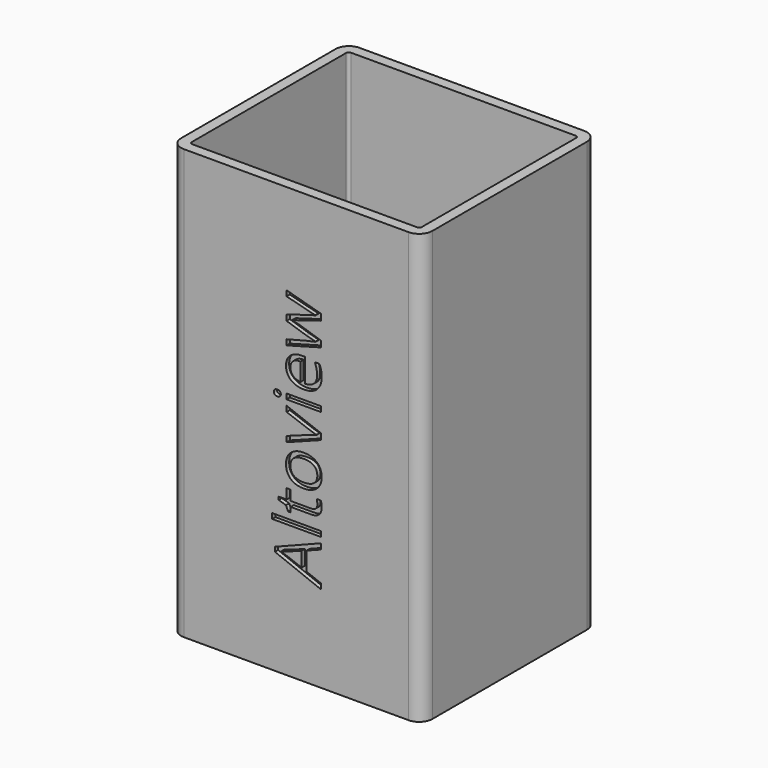
from build123d import *

# Parameters (mm, degrees)
F1_DEPTH     = 65
F2_T         = -1.6
F3_TEXT_SIZE = 9.7222222222
F4_DEPTH     = 0.6


# Not quite as in the source:
# - Text() gives the source's letters only with a copy of the font that has no kerning and outlines rounded to 1/6400 em; it was checked with that copy


with BuildPart() as f1:
    # F0 (on Top) → F1 (new body)
    with BuildSketch(Plane.XY):
        with BuildLine():
            Line((17, 16.6), (-17, 16.6))
            ThreePointArc((-17, 16.6), (-18.4142135624, 16.0142135624), (-19, 14.6))
            Line((-19, 14.6), (-19, -14.6))
            ThreePointArc((-19, -14.6), (-18.4142135624, -16.0142135624), (-17, -16.6))
            Line((-17, -16.6), (17, -16.6))
            ThreePointArc((17, -16.6), (18.4142135624, -16.0142135624), (19, -14.6))
            Line((19, -14.6), (19, 14.6))
            ThreePointArc((19, 14.6), (18.4142135624, 16.0142135624), (17, 16.6))
        make_face()
    extrude(amount=F1_DEPTH)

    # F2
    f2_openings = [f1.faces().sort_by_distance(p)[0] for p in [
        (0, 0, 65),
    ]]
    offset(amount=F2_T, openings=f2_openings)

    # F3 (on face) → F4 (cut)
    with BuildSketch(Plane.XZ.offset(16.6)):
        with Locations(Location((3.7543848261, 13.1056857639), (0, 0, 90))):
            Text('Altoview', F3_TEXT_SIZE, font='Open Sans', text_align=(TextAlign.LEFT, TextAlign.BOTTOM))
    extrude(amount=-F4_DEPTH, mode=Mode.SUBTRACT)


solid = f1.part
